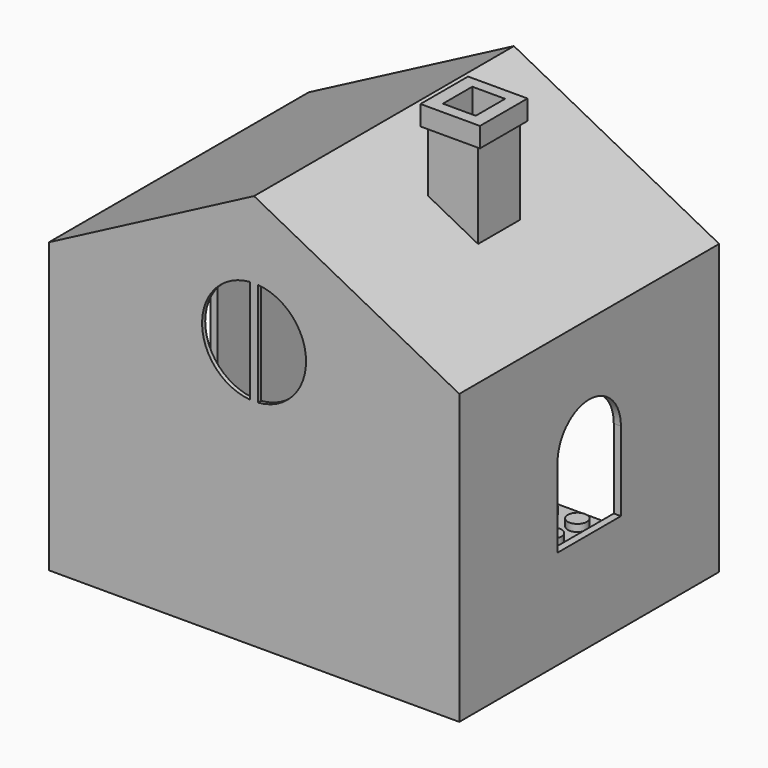
from build123d import *

# Parameters (mm, degrees)
F1_DEPTH  = 41
F3_DEPTH  = 25
F5_DEPTH  = 25
F7_DEPTH  = 40
F8_DEPTH  = 40
F10_R     = 2.4
F11_DEPTH = 1.8
F12_DEPTH = 25
F14_W     = 12.6157701015
F14_H     = 13.207135722
F14_W_2   = 8.2791037858
F14_H_2   = 9.2647057027
F14_W_3   = 15.008058399
F14_H_3   = 15.008058399
F16_DEPTH = 5
F18_DEPTH = 1
F19_R     = 5


# Not quite as in the source:
# - a feature names something its author has since deleted; it is built from what else it names


with BuildPart() as f1:
    # F0 (on Front) → F1 (new body, symmetric)
    with BuildSketch(Plane.XZ):
        Polygon((-51.8000006676, -1.8000006676), (0, -1.8000006676), (51.8000006676, -1.8000006676), (51.8000006676, 71.0895588475), (0, 98.1999993324), (-51.8000006676, 71.0895588475), align=None)
        Polygon((50, 0), (0, 0), (-50, 0), (-50, 70), (0, 96.1683785092), (50, 70), align=None, mode=Mode.SUBTRACT)
        Polygon((-50, 0), (0, 0), (50, 0), (50, 70), (0, 96.1683785092), (-50, 70), align=None)
    extrude(amount=F1_DEPTH, both=True)

    # F2 (on face) → F3 (cut)
    with BuildSketch(Plane(origin=(-51.8000006676, 0, 0), x_dir=(0, -1, 0), z_dir=(-1, 0, 0))):
        with BuildLine():
            Line((-10, 43.1999993324), (-10, 23.1999993324))
            Line((-10, 23.1999993324), (10, 23.1999993324))
            Line((10, 23.1999993324), (10, 43.1999993324))
            ThreePointArc((10, 43.1999993324), (0, 53.1999993324), (-10, 43.1999993324))
        make_face()
    extrude(amount=-F3_DEPTH, mode=Mode.SUBTRACT)

    # F4 (on face) → F5 (cut)
    with BuildSketch(Plane.YZ.offset(51.8000006676)):
        with BuildLine():
            Line((-10, 43.1999993324), (-10, 23.1999993324))
            Line((-10, 23.1999993324), (10, 23.1999993324))
            Line((10, 23.1999993324), (10, 43.1999993324))
            ThreePointArc((10, 43.1999993324), (0, 53.1999993324), (-10, 43.1999993324))
        make_face()
    extrude(amount=-F5_DEPTH, mode=Mode.SUBTRACT)

    # F0 (on Front) → F7 (cut)
    with BuildSketch(Plane.XZ):
        Polygon((-50, 0), (0, 0), (50, 0), (50, 70), (0, 96.1683785092), (-50, 70), align=None)
    extrude(amount=-F7_DEPTH, mode=Mode.SUBTRACT)

    # F0 (on Front) → F8 (cut)
    with BuildSketch(Plane.XZ):
        Polygon((-50, 0), (0, 0), (50, 0), (50, 70), (0, 96.1683785092), (-50, 70), align=None)
    extrude(amount=F8_DEPTH, mode=Mode.SUBTRACT)

    # F10 (on Top) → F11 (join)
    with BuildSketch(Plane.XY):
        with Locations((-44, 36)):
            Circle(F10_R)
        with Locations((-44, 28)):
            Circle(F10_R)
        with Locations((-44, 20)):
            Circle(F10_R)
        with Locations((-44, 12)):
            Circle(F10_R)
        with Locations((-44, 4)):
            Circle(F10_R)
        with Locations((-44, -4)):
            Circle(F10_R)
        with Locations((-44, -12)):
            Circle(F10_R)
        with Locations((-44, -20)):
            Circle(F10_R)
        with Locations((-44, -28)):
            Circle(F10_R)
        with Locations((-44, -36)):
            Circle(F10_R)
        with Locations((-36, 36)):
            Circle(F10_R)
        with Locations((-36, 28)):
            Circle(F10_R)
        with Locations((-36, 20)):
            Circle(F10_R)
        with Locations((-36, 12)):
            Circle(F10_R)
        with Locations((-36, 4)):
            Circle(F10_R)
        with Locations((-36, -4)):
            Circle(F10_R)
        with Locations((-36, -12)):
            Circle(F10_R)
        with Locations((-36, -20)):
            Circle(F10_R)
        with Locations((-36, -28)):
            Circle(F10_R)
        with Locations((-36, -36)):
            Circle(F10_R)
        with Locations((-28, 36)):
            Circle(F10_R)
        with Locations((-28, 28)):
            Circle(F10_R)
        with Locations((-28, 20)):
            Circle(F10_R)
        with Locations((-28, 12)):
            Circle(F10_R)
        with Locations((-28, 4)):
            Circle(F10_R)
        with Locations((-28, -4)):
            Circle(F10_R)
        with Locations((-28, -12)):
            Circle(F10_R)
        with Locations((-28, -20)):
            Circle(F10_R)
        with Locations((-28, -28)):
            Circle(F10_R)
        with Locations((-28, -36)):
            Circle(F10_R)
        with Locations((-20, 36)):
            Circle(F10_R)
        with Locations((-20, 28)):
            Circle(F10_R)
        with Locations((-20, 20)):
            Circle(F10_R)
        with Locations((-20, 12)):
            Circle(F10_R)
        with Locations((-20, 4)):
            Circle(F10_R)
        with Locations((-20, -4)):
            Circle(F10_R)
        with Locations((-20, -12)):
            Circle(F10_R)
        with Locations((-20, -20)):
            Circle(F10_R)
        with Locations((-20, -28)):
            Circle(F10_R)
        with Locations((-20, -36)):
            Circle(F10_R)
        with Locations((-12, 36)):
            Circle(F10_R)
        with Locations((-12, 28)):
            Circle(F10_R)
        with Locations((-12, 20)):
            Circle(F10_R)
        with Locations((-12, 12)):
            Circle(F10_R)
        with Locations((-12, 4)):
            Circle(F10_R)
        with Locations((-12, -4)):
            Circle(F10_R)
        with Locations((-12, -12)):
            Circle(F10_R)
        with Locations((-12, -20)):
            Circle(F10_R)
        with Locations((-12, -28)):
            Circle(F10_R)
        with Locations((-12, -36)):
            Circle(F10_R)
        with Locations((-4, 36)):
            Circle(F10_R)
        with Locations((-4, 28)):
            Circle(F10_R)
        with Locations((-4, 20)):
            Circle(F10_R)
        with Locations((-4, 12)):
            Circle(F10_R)
        with Locations((-4, 4)):
            Circle(F10_R)
        with Locations((-4, -4)):
            Circle(F10_R)
        with Locations((-4, -12)):
            Circle(F10_R)
        with Locations((-4, -20)):
            Circle(F10_R)
        with Locations((-4, -28)):
            Circle(F10_R)
        with Locations((-4, -36)):
            Circle(F10_R)
        with Locations((4, 36)):
            Circle(F10_R)
        with Locations((4, 28)):
            Circle(F10_R)
        with Locations((4, 20)):
            Circle(F10_R)
        with Locations((4, 12)):
            Circle(F10_R)
        with Locations((4, 4)):
            Circle(F10_R)
        with Locations((4, -4)):
            Circle(F10_R)
        with Locations((4, -12)):
            Circle(F10_R)
        with Locations((4, -20)):
            Circle(F10_R)
        with Locations((4, -28)):
            Circle(F10_R)
        with Locations((4, -36)):
            Circle(F10_R)
        with Locations((12, 36)):
            Circle(F10_R)
        with Locations((12, 28)):
            Circle(F10_R)
        with Locations((12, 20)):
            Circle(F10_R)
        with Locations((12, 12)):
            Circle(F10_R)
        with Locations((12, 4)):
            Circle(F10_R)
        with Locations((12, -4)):
            Circle(F10_R)
        with Locations((12, -12)):
            Circle(F10_R)
        with Locations((12, -20)):
            Circle(F10_R)
        with Locations((12, -28)):
            Circle(F10_R)
        with Locations((12, -36)):
            Circle(F10_R)
        with Locations((20, 36)):
            Circle(F10_R)
        with Locations((20, 28)):
            Circle(F10_R)
        with Locations((20, 20)):
            Circle(F10_R)
        with Locations((20, 12)):
            Circle(F10_R)
        with Locations((20, 4)):
            Circle(F10_R)
        with Locations((20, -4)):
            Circle(F10_R)
        with Locations((20, -12)):
            Circle(F10_R)
        with Locations((20, -20)):
            Circle(F10_R)
        with Locations((20, -28)):
            Circle(F10_R)
        with Locations((20, -36)):
            Circle(F10_R)
        with Locations((28, 36)):
            Circle(F10_R)
        with Locations((28, 28)):
            Circle(F10_R)
        with Locations((28, 20)):
            Circle(F10_R)
        with Locations((28, 12)):
            Circle(F10_R)
        with Locations((28, 4)):
            Circle(F10_R)
        with Locations((28, -4)):
            Circle(F10_R)
        with Locations((28, -12)):
            Circle(F10_R)
        with Locations((28, -20)):
            Circle(F10_R)
        with Locations((28, -28)):
            Circle(F10_R)
        with Locations((28, -36)):
            Circle(F10_R)
        with Locations((36, 36)):
            Circle(F10_R)
        with Locations((36, 28)):
            Circle(F10_R)
        with Locations((36, 20)):
            Circle(F10_R)
        with Locations((36, 12)):
            Circle(F10_R)
        with Locations((36, 4)):
            Circle(F10_R)
        with Locations((36, -4)):
            Circle(F10_R)
        with Locations((36, -12)):
            Circle(F10_R)
        with Locations((36, -20)):
            Circle(F10_R)
        with Locations((36, -28)):
            Circle(F10_R)
        with Locations((36, -36)):
            Circle(F10_R)
        with Locations((44, 36)):
            Circle(F10_R)
        with Locations((44, 28)):
            Circle(F10_R)
        with Locations((44, 20)):
            Circle(F10_R)
        with Locations((44, 12)):
            Circle(F10_R)
        with Locations((44, 4)):
            Circle(F10_R)
        with Locations((44, -4)):
            Circle(F10_R)
        with Locations((44, -12)):
            Circle(F10_R)
        with Locations((44, -20)):
            Circle(F10_R)
        with Locations((44, -28)):
            Circle(F10_R)
        with Locations((44, -36)):
            Circle(F10_R)
    extrude(amount=F11_DEPTH)

    # F9 (on face) → F12 (cut)
    with BuildSketch(Plane.XZ.offset(41)):
        with BuildLine():
            Line((-1, 52.6246078838), (-1, 78.8037083518))
            ThreePointArc((-1, 78.8037083518), (-13.1276930696, 65.7141581178), (-1, 52.6246078838))
        make_face()
        with BuildLine():
            ThreePointArc((1, 52.6246078838), (9.629746061, 56.7920330273), (13.1276930696, 65.7141581178))
            ThreePointArc((13.1276930696, 65.7141581178), (9.629746061, 74.6362832082), (1, 78.8037083518))
            Line((1, 78.8037083518), (1, 52.6246078838))
        make_face()
    extrude(amount=-F12_DEPTH, mode=Mode.SUBTRACT)

    # F14 (on offset) → F15 (join, up to the next surface of F1)
    with BuildSketch(Plane.XY.offset(110)):
        with Locations((22.7182414383, 0)):
            Rectangle(F14_W, F14_H)
        with Locations((22.7182414383, 0)):
            Rectangle(F14_W_2, F14_H_2, mode=Mode.SUBTRACT)
    extrude(until=Until.NEXT, dir=(0, 0, -1))

    # F14 (on offset) → F16 (join)
    with BuildSketch(Plane.XY.offset(110)):
        with Locations((22.7182414383, 0)):
            Rectangle(F14_W_3, F14_H_3)
        with Locations((22.7182414383, 0)):
            Rectangle(F14_W, F14_H, mode=Mode.SUBTRACT)
    extrude(amount=-F16_DEPTH)

    # F17 (on face) → F18 (cut)
    with BuildSketch(Plane(origin=(0, 41, 0), x_dir=(-1, 0, 0), z_dir=(0, 1, 0))):
        with BuildLine():
            Line((-45, 0), (45, 0))
            Line((45, 0), (45, 70))
            ThreePointArc((45, 70), (0, 85.0858858065), (-45, 70))
            Line((-45, 70), (-45, 0))
        make_face()
    extrude(amount=-F18_DEPTH, mode=Mode.SUBTRACT)

    # F19
    f19_edges = [f1.edges().sort_by_distance(p)[0] for p in [
        (45, 40.5, 70),
        (-45, 40.5, 70),
    ]]
    fillet(f19_edges, radius=F19_R)


solid = f1.part
